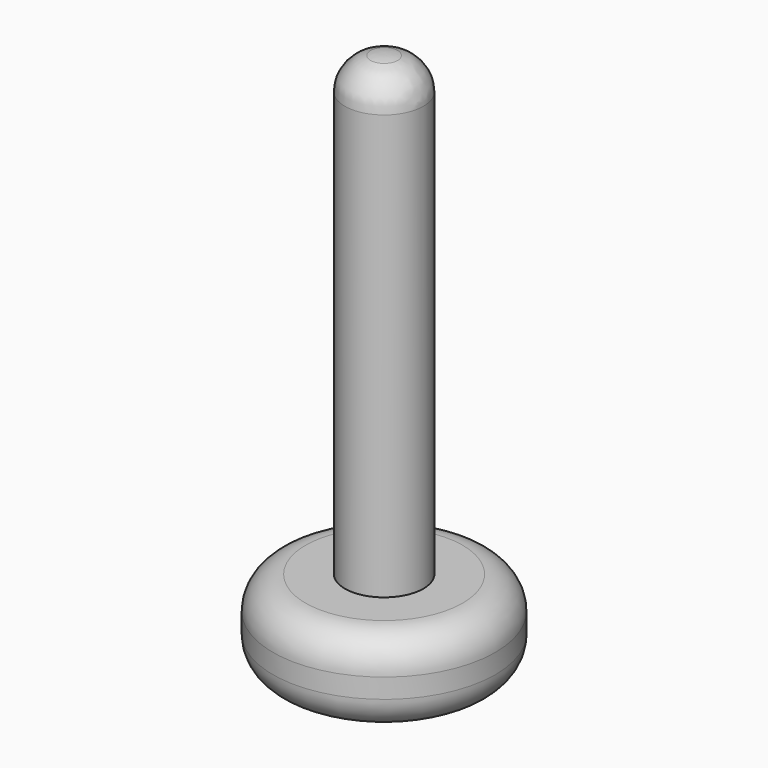
from build123d import *

# Parameters (mm, degrees)
F2_R         = 5
F3_R         = 5
F4_TEXT_SIZE = 15.3451601768
F5_DEPTH     = 0.75
F6_R         = 5


# Not quite as in the source:
# - Text() gives the source's letters only with a copy of the font that has no kerning and outlines rounded to 1/6400 em; it was checked with that copy


with BuildPart() as f1:
    # F0 (on Front) → F1 (revolve)
    with BuildSketch(Plane.XZ):
        with BuildLine():
            ThreePointArc((6, 80.7681679726), (3.2176955551, 82.4693311351), (0, 83))
            Line((0, 83), (0, 0))
            Line((0, 0), (17, 0))
            Line((17, 0), (17, 13))
            Line((17, 13), (6, 13))
            Line((6, 13), (6, 80.7681679726))
        make_face()
    revolve(axis=Axis((0, 0, 41.5), (0, 0, -1)))

    # F2
    f2_edges = [f1.edges().sort_by_distance(p)[0] for p in [
        (-17, 0, 13),
    ]]
    fillet(f2_edges, radius=F2_R)

    # F3
    f3_edges = [f1.edges().sort_by_distance(p)[0] for p in [
        (-17, 0, 0),
    ]]
    fillet(f3_edges, radius=F3_R)

    # F4 (on Top) → F5 (join, symmetric)
    with BuildSketch(Plane.XY):
        with Locations((-8.9001934975, -5.4219556041)):
            Text('TO', F4_TEXT_SIZE, font='Open Sans', font_style=FontStyle.ITALIC, text_align=(TextAlign.LEFT, TextAlign.BOTTOM))
    extrude(amount=F5_DEPTH, both=True)

    # F6
    f6_edges = [f1.edges().sort_by_distance(p)[0] for p in [
        (-6, 0, 80.768168),
    ]]
    fillet(f6_edges, radius=F6_R)


solid = f1.part
